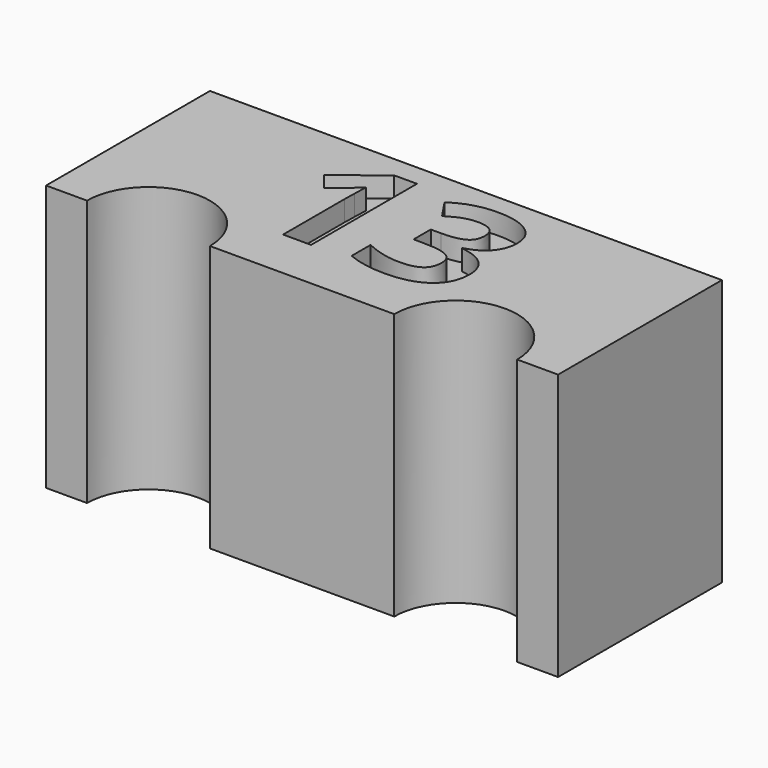
from build123d import *

# Parameters (mm, degrees)
F0_W         = 25
F0_H         = 10
F1_DEPTH     = 13
F2_R         = 3
F3_DEPTH     = 13.001
F4_TEXT_SIZE = 9.053372741
F5_DEPTH     = 1


# Not quite as in the source:
# - Text() gives the source's letters only with a copy of the font that has no kerning and outlines rounded to 1/6400 em; it was checked with that copy


with BuildPart() as f1:
    # F0 (on Top) → F1 (new body)
    with BuildSketch(Plane.XY):
        Rectangle(F0_W, F0_H)
    extrude(amount=F1_DEPTH)

    # F2 (on Top) → F3 (cut, through all)
    with BuildSketch(Plane.XY):
        with Locations((-7.5, -5)):
            Circle(F2_R)
        with Locations((7.5, -5)):
            Circle(F2_R)
    extrude(amount=F3_DEPTH, mode=Mode.SUBTRACT)

    # F4 (on face) → F5 (cut)
    with BuildSketch(Plane.XY.offset(13)):
        with Locations((-5.2863209271, -2.5184283736)):
            Text('13', F4_TEXT_SIZE, font='Open Sans', font_style=FontStyle.BOLD, text_align=(TextAlign.LEFT, TextAlign.BOTTOM))
    extrude(amount=-F5_DEPTH, mode=Mode.SUBTRACT)


solid = f1.part
